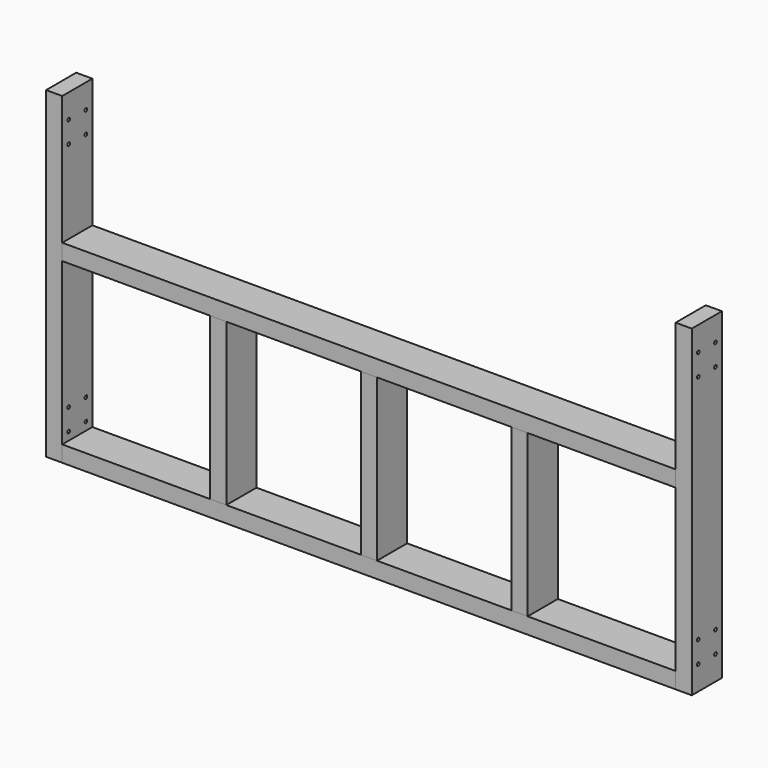
from build123d import *

# Parameters (mm, degrees)
F1_DEPTH = 762
F2_W     = 88.9
F2_H     = 38.1
F3_DEPTH = 1447.8
F4_W     = 38.1
F4_H     = 88.9
F5_DEPTH = 381
F6_R     = 3.96875
F7_DEPTH = 1524.001


with BuildPart() as f1:
    # F0 (on Top) → F1 (new body)
    with BuildSketch(Plane.XY):
        Polygon((-723.9, 0), (-723.9, 44.45), (-762, 44.45), (-762, -44.45), (-723.9, -44.45), align=None)
    extrude(amount=F1_DEPTH)


with BuildPart() as f1b:
    # F0 (on Top) → F1, piece 2 (new body)
    with BuildSketch(Plane.XY):
        Polygon((723.9, 44.45), (723.9, 0), (723.9, -44.45), (762, -44.45), (762, 44.45), align=None)
    extrude(amount=F1_DEPTH)


with BuildPart() as f3:
    # F2 (on face) → F3 (new body, through all)
    with BuildSketch(Plane.YZ.offset(-723.9)):
        with Locations((0, 19.05)):
            Rectangle(F2_W, F2_H)
    extrude(amount=F3_DEPTH)


with BuildPart() as f3b:
    # F2 (on face) → F3, piece 2 (new body, through all)
    with BuildSketch(Plane.YZ.offset(-723.9)):
        with Locations((0, 438.15)):
            Rectangle(F2_W, F2_H)
    extrude(amount=F3_DEPTH)


with BuildPart() as f5:
    # F4 (on face) → F5 (new body, through all)
    with BuildSketch(Plane.XY.offset(38.1)):
        Rectangle(F4_W, F4_H)
    extrude(amount=F5_DEPTH)


with BuildPart() as f5b:
    # F4 (on face) → F5, piece 2 (new body, through all)
    with BuildSketch(Plane.XY.offset(38.1)):
        with Locations((-355.6, 0)):
            Rectangle(F4_W, F4_H)
    extrude(amount=F5_DEPTH)


with BuildPart() as f5c:
    # F4 (on face) → F5, piece 3 (new body, through all)
    with BuildSketch(Plane.XY.offset(38.1)):
        with Locations((355.6, 0)):
            Rectangle(F4_W, F4_H)
    extrude(amount=F5_DEPTH)


with BuildPart() as f7_tool:
    # F6 (on face) → F7 (new body, through all)
    with BuildSketch(Plane(origin=(-762, 0, 0), x_dir=(0, -1, 0), z_dir=(-1, 0, 0))):
        with Locations((-25.4, 57.15)):
            Circle(F6_R)
        with Locations((-25.4, 107.95)):
            Circle(F6_R)
        with Locations((25.4, 107.95)):
            Circle(F6_R)
        with Locations((25.4, 57.15)):
            Circle(F6_R)
        with Locations((-25.4, 654.05)):
            Circle(F6_R)
        with Locations((-25.4, 704.85)):
            Circle(F6_R)
        with Locations((25.4, 704.85)):
            Circle(F6_R)
        with Locations((25.4, 654.05)):
            Circle(F6_R)
    extrude(amount=-F7_DEPTH)


with BuildPart() as f1_1:
    add(f1.part)

    # F7: cut by f7_tool
    add(f7_tool.part, mode=Mode.SUBTRACT)


with BuildPart() as f1b_1:
    add(f1b.part)

    # F7: cut by f7_tool
    add(f7_tool.part, mode=Mode.SUBTRACT)


solid = Compound([f3.part, f3b.part, f5.part, f5b.part, f5c.part, f1_1.part, f1b_1.part])
